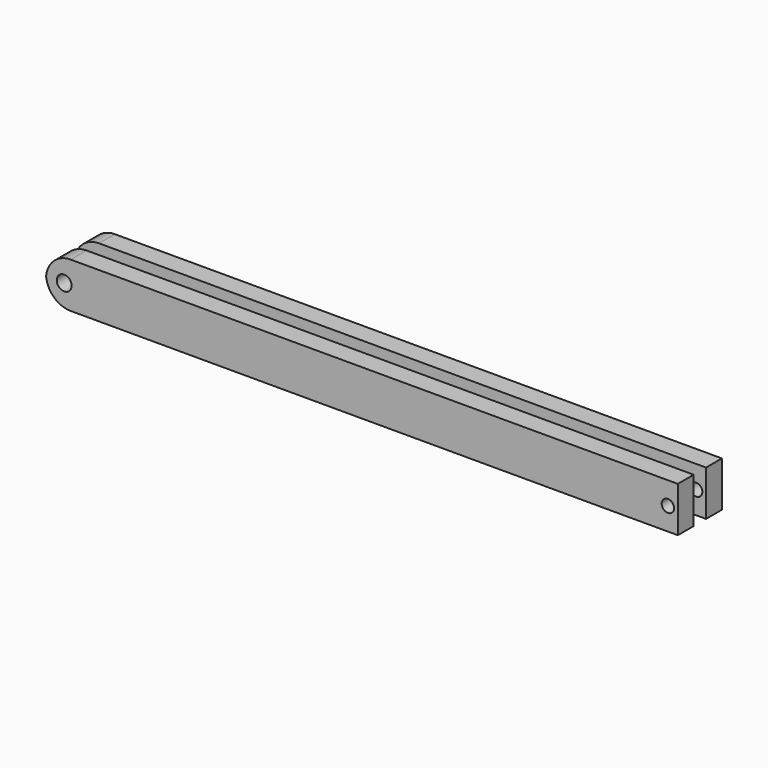
from build123d import *

# Parameters (mm, degrees)
F0_W        = 129.5146
F0_H        = 11.303
F1_DEPTH    = 9.271
F2_W        = 206.3660303733
F2_H        = 3.175
F3_DEPTH    = 7.5438
F4_W        = 3.7084
F4_H        = 3.175
F5_DEPTH    = 25.4
F6_W        = 16.3322
F6_H        = 3.175
F7_DEPTH    = 25.4
F8_T1_DEPTH = 29.464
F8_T3_DEPTH = 29.464
F9_R        = 1.524
F10_DEPTH   = 25.4
F12_DEPTH   = 25.4
F13_W       = 11.2141259015
F13_H       = 1.2269735361
F14_DEPTH   = 4.1656
F15_DEPTH   = 0.254
F16_DEPTH   = 3.175
F16_FACE_W  = 4.4019735361
F16_FACE_H  = 4.1656
F17_ANGLE   = 90


# Not quite as in the source:
# - a fillet or chamfer that OpenCascade refuses, or shapes differently, is made with other operations: its cross-section is extruded or revolved along the edge and cut away or added


with BuildPart() as f1:
    # F0 (on Top) → F1 (new body)
    with BuildSketch(Plane.XY):
        Rectangle(F0_W, F0_H)
    extrude(amount=F1_DEPTH)

    # F2 (on face) → F3 (cut)
    with BuildSketch(Plane.XY.offset(9.271)):
        Rectangle(F2_W, F2_H)
    extrude(amount=-F3_DEPTH, mode=Mode.SUBTRACT)

    # F4 (on face) → F5 (cut)
    with BuildSketch(Plane.XY.offset(1.7272)):
        with Locations((62.9031, 0)):
            Rectangle(F4_W, F4_H)
    extrude(amount=-F5_DEPTH, mode=Mode.SUBTRACT)

    # F6 (on face) → F7 (cut)
    with BuildSketch(Plane.XY.offset(1.7272)):
        with Locations((-56.5912, 0)):
            Rectangle(F6_W, F6_H)
    extrude(amount=-F7_DEPTH, mode=Mode.SUBTRACT)

    # F8: fillet of radius 5.08 on 4 edges, made by hand

    # F8_s2 → F8_t1 (cut)
    with BuildSketch(Plane.XZ.offset(-11.1125)):
        with BuildLine():
            ThreePointArc((-64.7573, 4.191), (-63.2694024484, 7.7831024484), (-59.6773, 9.271))
            Line((-59.6773, 9.271), (-64.7573, 9.271))
            Line((-64.7573, 9.271), (-64.7573, 4.191))
        make_face()
        with BuildLine():
            ThreePointArc((-64.7573, 5.08), (-63.2694024484, 1.4878975516), (-59.6773, 0))
            Line((-59.6773, 0), (-64.7573, 0))
            Line((-64.7573, 0), (-64.7573, 5.08))
        make_face()
    extrude(amount=F8_T1_DEPTH, mode=Mode.SUBTRACT)

    # F8_s4 → F8_t3 (cut)
    with BuildSketch(Plane.XZ.offset(-18.3515)):
        with BuildLine():
            ThreePointArc((-59.6773, 9.271), (-63.2694024484, 7.7831024484), (-64.7573, 4.191))
            Line((-64.7573, 4.191), (-64.7573, 9.271))
            Line((-64.7573, 9.271), (-59.6773, 9.271))
        make_face()
        with BuildLine():
            ThreePointArc((-64.7573, 5.08), (-63.2694024484, 1.4878975516), (-59.6773, 0))
            Line((-59.6773, 0), (-64.7573, 0))
            Line((-64.7573, 0), (-64.7573, 5.08))
        make_face()
    extrude(amount=F8_T3_DEPTH, mode=Mode.SUBTRACT)

    # F9 (on face) → F10 (cut)
    with BuildSketch(Plane.XZ.offset(5.6515)):
        with Locations((-61.0294157593, 4.6167229302)):
            Circle(F9_R)
    extrude(amount=-F10_DEPTH, mode=Mode.SUBTRACT)

    # F11 (on face) → F12 (cut)
    with BuildSketch(Plane.XZ.offset(5.6515)):
        with BuildLine():
            Line((61.4553, 4.6355), (63.9953, 4.6355))
            ThreePointArc((63.9953, 4.6355), (62.7253, 5.9055), (61.4553, 4.6355))
        make_face()
        with BuildLine():
            ThreePointArc((61.4553, 4.6355), (62.7253, 3.3655), (63.9953, 4.6355))
            Line((63.9953, 4.6355), (61.4553, 4.6355))
        make_face()
    extrude(amount=-F12_DEPTH, mode=Mode.SUBTRACT)


with BuildPart() as f14:
    # F13 (on Top) → F14 (new body)
    with BuildSketch(Plane.XY):
        with Locations((67.7984524518, -0.613486768)):
            Rectangle(F13_W, F13_H)
    extrude(amount=F14_DEPTH)


with BuildPart() as f15:
    # F15 (new): a face of the model
    f15_faces = [f14.part.faces().sort_by_distance(p)[0] for p in [
        (73.4055154026, -0.613486768, 2.0828),
    ]]
    extrude(f15_faces, amount=F15_DEPTH)


with BuildPart() as f14_1:
    add(f14.part)

    # F16 (add): a face of the model
    f16_faces = [f15.part.faces().sort_by_distance(p)[0] for p in [
        (73.5325154026, -1.2269735361, 2.0828),
    ]]

    add(f15.part)  # F16 merges F15
    extrude(f16_faces, amount=F16_DEPTH)


with BuildPart() as f17:
    # F16_face (on face) → F17 (revolve)
    with BuildSketch(Plane(origin=(73.6595154026, -2.200986768, 2.0828), x_dir=(0, 1, 0), z_dir=(1, 0, 0))):
        Rectangle(F16_FACE_W, F16_FACE_H)
    revolve(axis=Axis((73.6595154026, -2.200986768, 0), (0, -1, 0)), revolution_arc=F17_ANGLE)


with BuildPart() as f18_1:
    # F18: instance of F14
    add(f14_1.part.mirror(Plane.XZ))


with BuildPart() as f18_2:
    # F18: instance of F17
    add(f17.part.mirror(Plane.XZ))


solid = f1.part
